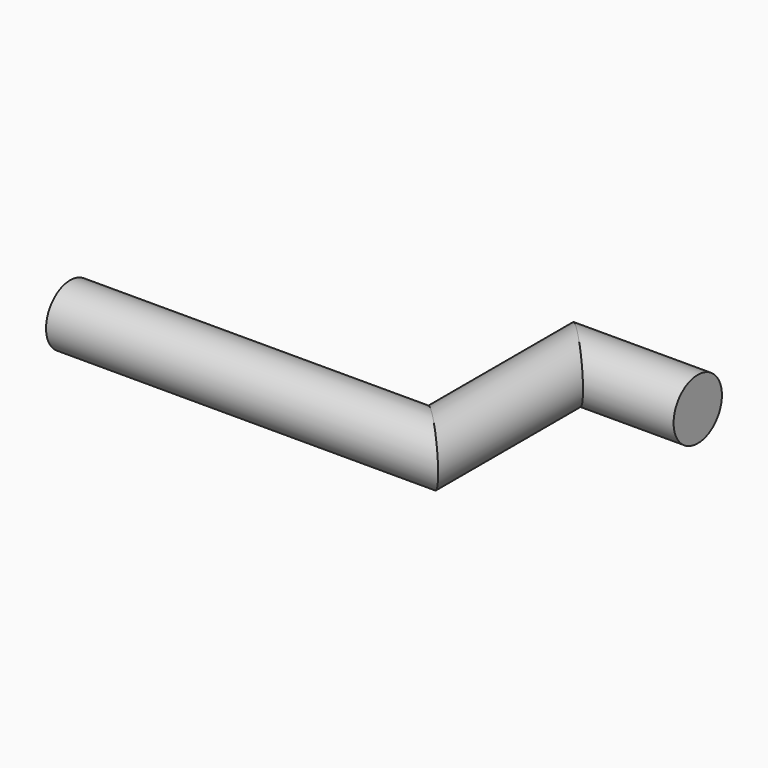
from build123d import *

# Parameters (mm, degrees)
F1_R = 3.1786059016


with BuildPart() as f2:
    # F2: sweep along a path in F0
    with BuildLine(Plane.XY) as f2_path:
        Line((0, 30.4371919483), (-12.6951197162, 30.4371919483))
        Line((-12.6951197162, 30.4371919483), (-12.6951197162, 11.3803073764))
        Line((-12.6951197162, 11.3803073764), (-50.7885627449, 11.3803073764))
    # F1 (on Right) → F2 (sweep)
    with BuildSketch(Plane.YZ):
        with Locations((30.454127118, 0)):
            Circle(F1_R)
    sweep(path=f2_path.line, transition=Transition.RIGHT)


solid = f2.part
